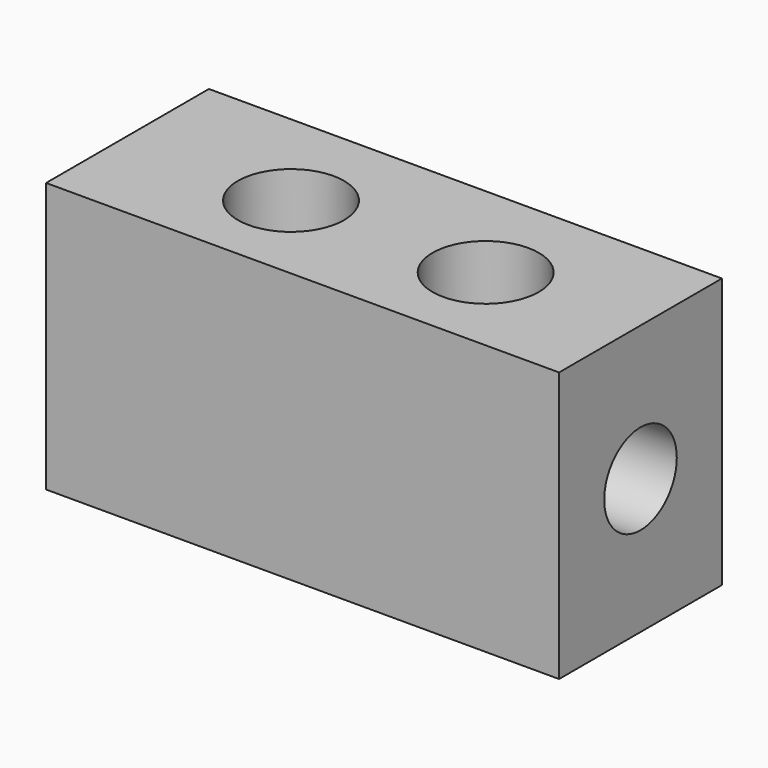
from build123d import *

# Parameters (mm, degrees)
F0_W     = 711.2
F0_H     = 387.35
F1_DEPTH = 292.1
F2_R     = 65.0875
F3_DEPTH = 375
F4_R     = 76.219
F5_DEPTH = 388
F7_DEPTH = 25


with BuildPart() as f1:
    # F0 (on Front) → F1 (new body)
    with BuildSketch(Plane.XZ):
        Rectangle(F0_W, F0_H)
    extrude(amount=-F1_DEPTH)

    # F2 (on Right) → F3 (cut, symmetric)
    with BuildSketch(Plane.YZ):
        with Locations((146.05, 0)):
            Circle(F2_R)
    extrude(amount=F3_DEPTH, both=True, mode=Mode.SUBTRACT)

    # F4 (on face) → F5 (cut)
    with BuildSketch(Plane.XY.offset(193.675)):
        with Locations((139.7, 138.176)):
            Circle(F4_R)
        with Locations((-139.7, 138.176)):
            Circle(F4_R)
    extrude(amount=-F5_DEPTH, mode=Mode.SUBTRACT)

    # F7 (add): a face of the model
    f7_faces = [f1.faces().sort_by_distance(p)[0] for p in [
        (-355.6, 146.05, 188.823583377),
    ]]
    extrude(f7_faces, amount=F7_DEPTH)


solid = f1.part
